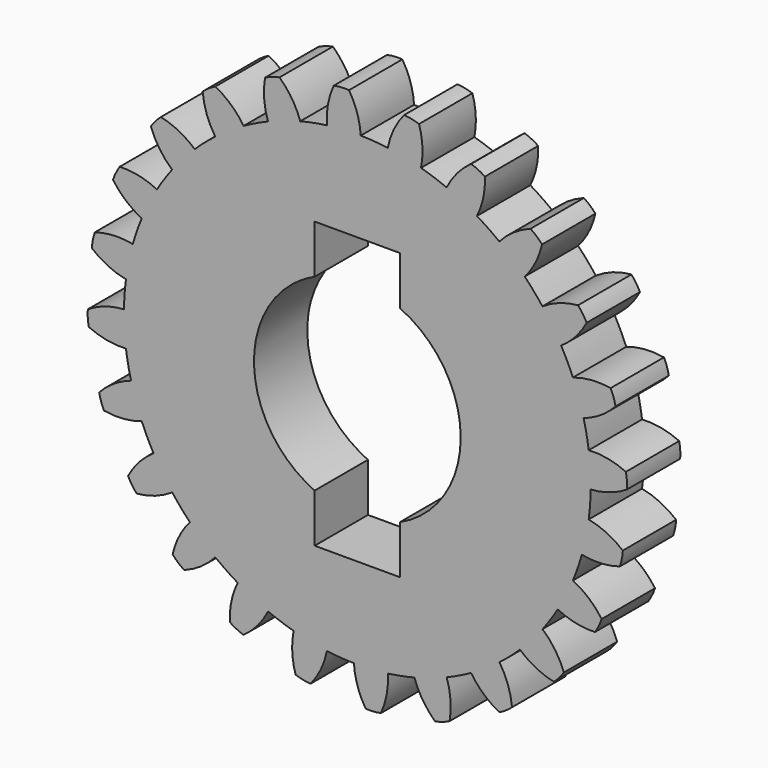
from build123d import *

# Parameters (mm, degrees)
F1_DEPTH = 12.7
F2_COUNT = 24
F2_ANGLE = 345
F3_DEPTH = 25.4


# Not quite as in the source:
# - a feature names something its author has since deleted; it is built from what else it names


with BuildPart() as f1:
    # F0 (on Front) → F1 (new body)
    with BuildSketch(Plane.XZ):
        with BuildLine():
            ThreePointArc((-5.81118052, 44.0684998719), (-29.3043983549, -33.4223688128), (44.45, 0))
            ThreePointArc((44.45, 0), (31.6596085179, 31.2005078243), (0.6492491116, 44.4452581902))
            ThreePointArc((0.6492491116, 44.4452581902), (-2.5878312685, 44.3746056808), (-5.81118052, 44.0684998719))
        make_face()
        with BuildLine():
            ThreePointArc((8.128, 17.9286039892), (16.5453755624, 10.6653538385), (19.685, 0))
            ThreePointArc((19.685, 0), (16.5453755624, -10.6653538385), (8.128, -17.9286039892))
            Line((8.128, -17.9286039892), (8.128, -27.178))
            Line((8.128, -27.178), (-8.128, -27.178))
            Line((-8.128, -27.178), (-8.128, -17.9286039892))
            ThreePointArc((-8.128, -17.9286039892), (-19.685, 0), (-8.128, 17.9286039892))
            Line((-8.128, 17.9286039892), (-8.128, 27.178))
            Line((-8.128, 27.178), (8.128, 27.178))
            Line((8.128, 27.178), (8.128, 17.9286039892))
        make_face(mode=Mode.SUBTRACT)
        with BuildLine():
            ThreePointArc((-5.81118052, 44.0684998719), (-2.5878312685, 44.3746056808), (0.6492491116, 44.4452581902))
            ThreePointArc((0.6492491116, 44.4452581902), (-0.0343594341, 48.0324601777), (-1.5864878253, 51.3379459514))
            ThreePointArc((-1.5864878253, 51.3379459514), (-3.0455527066, 51.3454237754), (-4.4911590337, 51.147563742))
            ThreePointArc((-4.4911590337, 51.147563742), (-5.5943052126, 47.6906625485), (-5.81118052, 44.0684998719))
        make_face()
    extrude(amount=F1_DEPTH)

    # F2: F1 ×24 about axis
    f2_axis = Axis((0, 0, 0), (0, 1, 0))


with BuildPart() as f1_1:
    add(f1.part)
    for i in range(1, F2_COUNT):
        add(f1.part.rotate(f2_axis, i * F2_ANGLE / (F2_COUNT - 1)))


with BuildPart() as f3:
    # F0 (on Front) → F3 (new body, symmetric)
    with BuildSketch(Plane.XZ):
        with BuildLine():
            ThreePointArc((-8.128, 17.9286039892), (0, 19.685), (8.128, 17.9286039892))
            Line((8.128, 17.9286039892), (8.128, 27.178))
            Line((8.128, 27.178), (-8.128, 27.178))
            Line((-8.128, 27.178), (-8.128, 17.9286039892))
        make_face()
    extrude(amount=F3_DEPTH, both=True)


with BuildPart() as f3b:
    # F0 (on Front) → F3, piece 2 (new body, symmetric)
    with BuildSketch(Plane.XZ):
        with BuildLine():
            Line((8.128, -27.178), (8.128, -17.9286039892))
            ThreePointArc((8.128, -17.9286039892), (0, -19.685), (-8.128, -17.9286039892))
            Line((-8.128, -17.9286039892), (-8.128, -27.178))
            Line((-8.128, -27.178), (8.128, -27.178))
        make_face()
    extrude(amount=F3_DEPTH, both=True)


with BuildPart() as f1_2:
    add(f1_1.part)

    # F4: cut F3, F3b
    add(f3.part, mode=Mode.SUBTRACT)
    add(f3b.part, mode=Mode.SUBTRACT)


solid = f1_2.part
